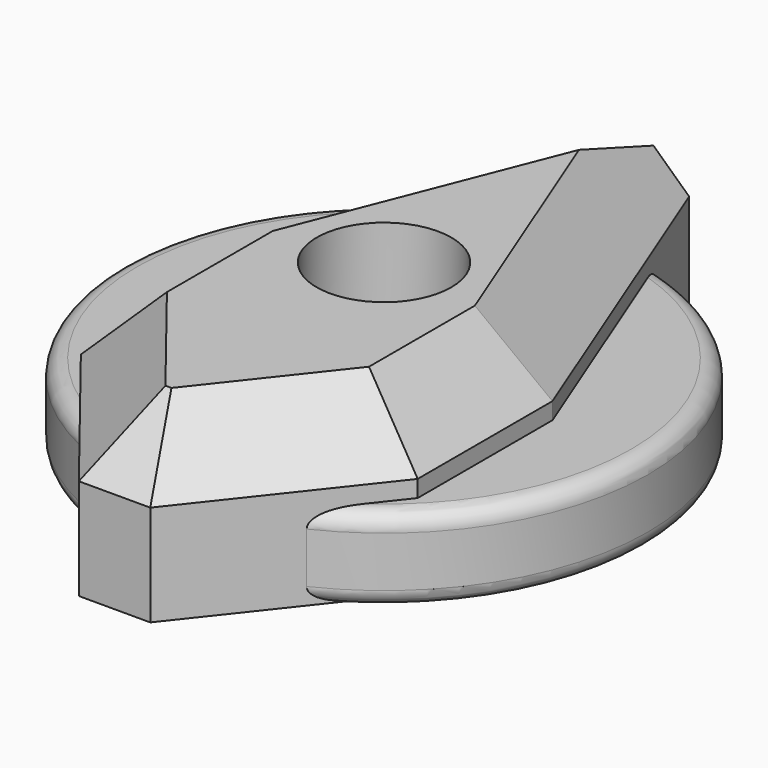
from build123d import *

# Parameters (mm, degrees)
F0_W         = 25.4
F0_H         = 50.8
F0_R         = 5.08
F1_DEPTH     = 12.7
F3_DEPTH     = 25.4
F4_T1_DEPTH  = 47.9732038629
F4_T3_DEPTH  = 31.5130991577
F4_T5_DEPTH  = 42.2974691352
F4_T7_DEPTH  = 42.2974691352
F4_T9_DEPTH  = 62.5709452641
F4_T11_DEPTH = 62.5736078482
F4_T16_DEPTH = 31.520364883
F4_T21_DEPTH = 31.520364883
F5_R         = 19.9015863144
F6_DEPTH     = 6.35
F7_R         = 1.27


# Not quite as in the source:
# - a fillet or chamfer that OpenCascade refuses, or shapes differently, is made with other operations: its cross-section is extruded or revolved along the edge and cut away or added


with BuildPart() as f1:
    # F0 (on Top) → F1 (new body)
    with BuildSketch(Plane.XY):
        Rectangle(F0_W, F0_H)
        Circle(F0_R, mode=Mode.SUBTRACT)
    extrude(amount=F1_DEPTH)

    # F2 (on face) → F3 (cut)
    with BuildSketch(Plane.XY.offset(12.7)):
        Polygon((-12.7, 25.4), (-12.7, 0), (-2.6996657252, 25.4), align=None)
        Polygon((-2.6924, -25.4), (-12.7, -12.7), (-12.7, -25.4), align=None)
        Polygon((12.7, -12.7), (2.6924, -25.4), (12.7, -25.4), align=None)
        Polygon((12.7, 25.4), (2.6924, 25.4), (12.7, 0), align=None)
    extrude(amount=-F3_DEPTH, mode=Mode.SUBTRACT)

    # F4: chamfer of 5.08 on 8 edges, made by hand

    # F4_s2 → F4_t1 (cut)
    with BuildSketch(Plane.XZ.offset(-22.2090542841)):
        Polygon((-7.62, 12.7), (-12.7, 7.62), (-12.7, 12.7), align=None)
        Polygon((12.7, 7.62), (7.62, 12.7), (12.7, 12.7), align=None)
    extrude(amount=F4_T1_DEPTH, mode=Mode.SUBTRACT)

    # F4_s4 → F4_t3 (cut)
    with BuildSketch(Plane.YZ.offset(-15.7565495789)):
        Polygon((-20.32, 12.7), (-25.4, 7.62), (-25.4, 12.7), align=None)
    extrude(amount=F4_T3_DEPTH, mode=Mode.SUBTRACT)

    # F4_s6 → F4_t5 (cut)
    with BuildSketch(Plane(origin=(6.7769328826, 8.6001686327, 0), x_dir=(0, 0, 1), z_dir=(-0.6189309664, -0.7854453888, 0))):
        Polygon((12.7, -12.7555797114), (7.62, -17.8355797114), (12.7, -17.8355797114), align=None)
    extrude(amount=F4_T5_DEPTH, mode=Mode.SUBTRACT)

    # F4_s8 → F4_t7 (cut)
    with BuildSketch(Plane(origin=(19.4022805654, -24.6221834587, 0), x_dir=(0, 0, 1), z_dir=(-0.6189309664, 0.7854453888, 0))):
        Polygon((12.7, -12.7555797114), (7.62, -17.8355797114), (12.7, -17.8355797114), align=None)
    extrude(amount=F4_T7_DEPTH, mode=Mode.SUBTRACT)

    # F4_s10 → F4_t9 (cut)
    with BuildSketch(Plane(origin=(-9.8405603892, -24.994187896, 0), x_dir=(0, 0, 1), z_dir=(0.3663429193, 0.9304799114, 0))):
        Polygon((12.7, -6.7370948746), (7.62, -11.8170948746), (12.7, -11.8170948746), align=None)
    extrude(amount=F4_T9_DEPTH, mode=Mode.SUBTRACT)

    # F4_s12 → F4_t11 (cut)
    with BuildSketch(Plane(origin=(-13.0899935353, 33.2233338458, 0), x_dir=(0, 0, 1), z_dir=(0.36657333, -0.9303891625, 0))):
        Polygon((7.62, -11.8159423639), (12.7, -6.7359423639), (12.7, -11.8159423639), align=None)
    extrude(amount=F4_T11_DEPTH, mode=Mode.SUBTRACT)


with BuildPart() as f4_tool14:
    # F4_s15 → F4_t16 (new body)
    with BuildSketch(Plane.YZ.offset(15.7565495789)):
        Polygon((20.32, 12.7), (25.4, 7.62), (25.4, 12.7), align=None)
    extrude(amount=-F4_T16_DEPTH)

    split(bisect_by=Plane(origin=(9.0414950692, 3.5623490573, 9.7179711819), x_dir=(-0.36657333, 0.9303891625, 0), z_dir=(0.657884486, 0.2592064875, 0.7071067812)), keep=Keep.TOP)


with BuildPart() as f1_1:
    add(f1.part)

    # F4_t13: cut F4_tool14
    add(f4_tool14.part, mode=Mode.SUBTRACT)


with BuildPart() as f4_tool19:
    # F4_s20 → F4_t21 (new body)
    with BuildSketch(Plane.YZ.offset(15.7565495789)):
        Polygon((20.32, 12.7), (25.4, 7.62), (25.4, 12.7), align=None)
    extrude(amount=-F4_T21_DEPTH)

    split(bisect_by=Plane(origin=(-9.0429131582, 3.5603210394, 9.7185474373), x_dir=(-0.3663429193, -0.9304799114, 0), z_dir=(-0.6579486551, 0.2590435625, 0.7071067812)), keep=Keep.TOP)


with BuildPart() as f1_2:
    add(f1_1.part)

    # F4_t18: cut F4_tool19
    add(f4_tool19.part, mode=Mode.SUBTRACT)

    # F5 (on Top) → F6 (join)
    with BuildSketch(Plane.XY):
        Circle(F5_R)
    extrude(amount=F6_DEPTH)

    # F7
    f7_edges = [f1_2.edges().sort_by_distance(p)[0] for p in [
        (19.817994, 1.822158, 0),
        (19.817994, 1.822158, 6.35),
        (-19.818285, 1.818991, 6.35),
        (-19.818285, 1.818991, 0),
    ]]
    fillet(f7_edges, radius=F7_R)


solid = f1_2.part
